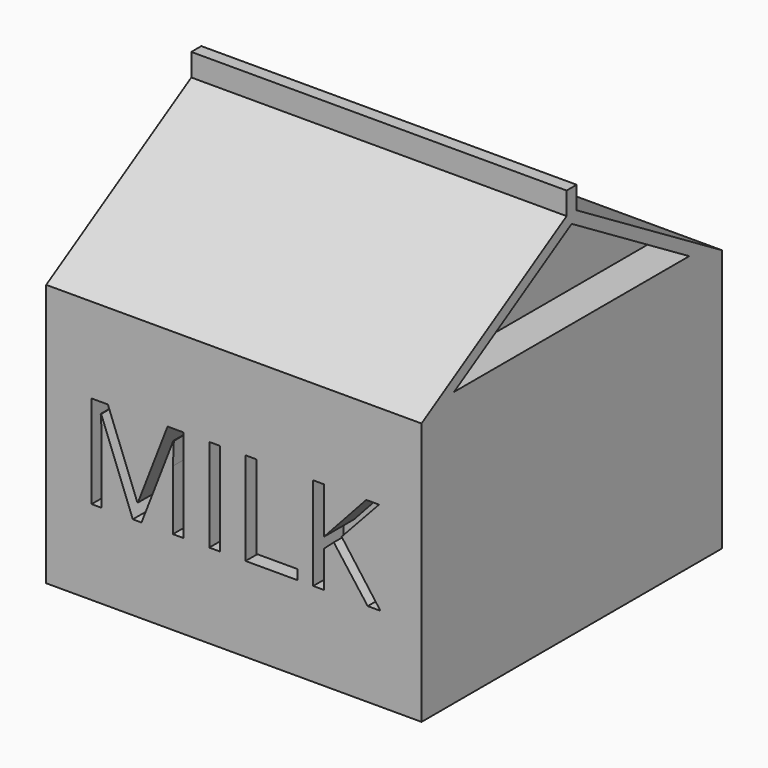
from build123d import *

# Parameters (mm, degrees)
F0_W         = 10
F0_H         = 10
F1_DEPTH     = 7
F3_DEPTH     = 10
F5_DEPTH     = 25
F6_DEPTH     = 0.6
F8_DEPTH     = 9
F9_DEPTH     = 1
F7_TEXT_SIZE = 3.4722222222
F10_DEPTH    = 1


# Not quite as in the source:
# - Text() gives the source's letters only with a copy of the font that has no kerning and outlines rounded to 1/6400 em; it was checked with that copy


with BuildPart() as f1:
    # F0 (on Top) → F1 (new body)
    with BuildSketch(Plane.XY):
        with Locations((-5, 5)):
            Rectangle(F0_W, F0_H)
    extrude(amount=F1_DEPTH)

    # F2 (on face) → F3 (join)
    with BuildSketch(Plane.YZ):
        Polygon((5.1677079975, 9.8993752015), (4.8322920025, 9.8993752015), (0, 7), (10, 7), align=None)
    extrude(amount=-F3_DEPTH)

    # F4 (on face) → F5 (cut)
    with BuildSketch(Plane.YZ):
        Polygon((8.9169048105, 7.3), (5, 9.6501428863), (1.0830951895, 7.3), align=None)
    extrude(amount=-F5_DEPTH, mode=Mode.SUBTRACT)

    # F6 (add): a face of the model
    f6_faces = [f1.faces().sort_by_distance(p)[0] for p in [
        (-5, 5, 9.8993752015),
    ]]
    extrude(f6_faces, amount=F6_DEPTH)

    # F4 (on face) → F8 (join)
    with BuildSketch(Plane.YZ):
        Polygon((8.9169048105, 7.3), (5, 9.6501428863), (1.0830951895, 7.3), align=None)
    extrude(amount=-F8_DEPTH)

    # F4 (on face) → F9 (cut)
    with BuildSketch(Plane.YZ):
        Polygon((8.9169048105, 7.3), (5, 9.6501428863), (1.0830951895, 7.3), align=None)
    extrude(amount=-F9_DEPTH, mode=Mode.SUBTRACT)

    # F7 (on face) → F10 (cut)
    with BuildSketch(Plane.XZ):
        with Locations((-9.1311762153, 2.25)):
            Text('MILK', F7_TEXT_SIZE, font='Open Sans', text_align=(TextAlign.LEFT, TextAlign.BOTTOM))
    extrude(amount=-F10_DEPTH, mode=Mode.SUBTRACT)


solid = f1.part
